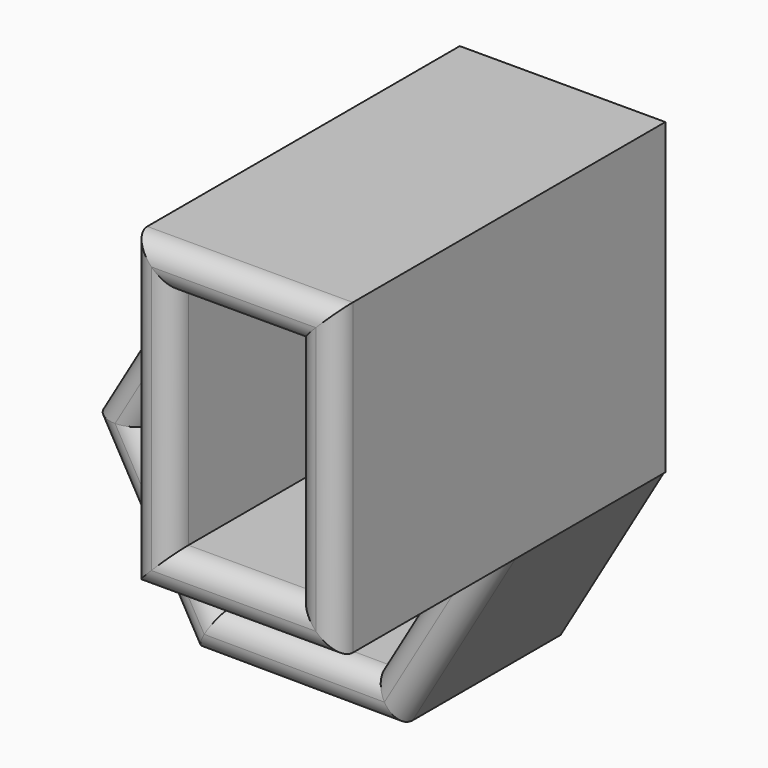
from build123d import *

# Parameters (mm, degrees)
F1_DEPTH = 101.6
F2_DEPTH = 50.8
F3_T     = -10.16
F4_R     = 5.07999


# Not quite as in the source:
# - a fillet or chamfer is up to 0.001 mm smaller than in the source, because OpenCascade refuses the exact size


with BuildPart() as f1:
    # F0 (on Front) → F1 (new body)
    with BuildSketch(Plane.XZ):
        Polygon((0, 43.6448735309), (0, 0), (50.223051581, 0), (50.8, 0), (50.8, 76.2), (0, 76.2), align=None)
    extrude(amount=F1_DEPTH)

    # F0 (on Front) → F2 (join)
    with BuildSketch(Plane.XZ):
        Polygon((50.223051581, 0), (0, 0), (0, 43.6448735309), (-24.9360222917, 43.7942571525), (-50.3949503798, 0.3018998023), (-25.4589280881, -43.4923573502), (24.9360222917, -43.7942571525), (50.3949503798, -0.3018998023), align=None)
    extrude(amount=F2_DEPTH)

    # F3: a shell. OpenCascade refuses it in one call, so the cavity is built on its own and cut out:
    # the body offset inwards by the wall thickness, plus a prism from it out through each open face.
    f3_core = offset(f1.part, amount=F3_T, kind=Kind.INTERSECTION, mode=Mode.PRIVATE)
    f3_exits = [f3_core.faces().sort_by_distance(p)[0] for p in [
        (25.4, -91.44, 38.1),
        (-1.965126, -40.64, -2.131269),
    ]]
    add(f3_core, mode=Mode.SUBTRACT)
    extrude(f3_exits, amount=-F3_T, mode=Mode.SUBTRACT)

    # F4 (radius 5.08 in the source; OpenCascade refuses exactly that, so slightly less here)
    f4_edges = [f1.edges().sort_by_distance(p)[0] for p in [
        (25.4, -101.6, 66.04),
        (40.64, -101.6, 38.1),
        (25.4, -101.6, 10.16),
        (10.16, -101.6, 38.1),
        (-28.897258, -50.8, 16.91546),
        (-29.097847, -50.8, -16.56803),
        (-0.200589, -50.8, -33.48349),
        (28.897258, -50.8, -16.91546),
        (-12.468011, -50.8, 43.719565),
        (-37.665486, -50.8, 22.048078),
        (-37.926939, -50.8, -21.595229),
        (-0.261453, -50.8, -43.643307),
        (37.665486, -50.8, -22.048078),
        (0, -101.6, 38.1),
        (25.4, -101.6, 76.2),
        (50.8, -101.6, 38.1),
        (25.4, -101.6, 0),
        (-9.565556, -50.8, 33.541995),
    ]]
    fillet(f4_edges, radius=F4_R)


solid = f1.part
